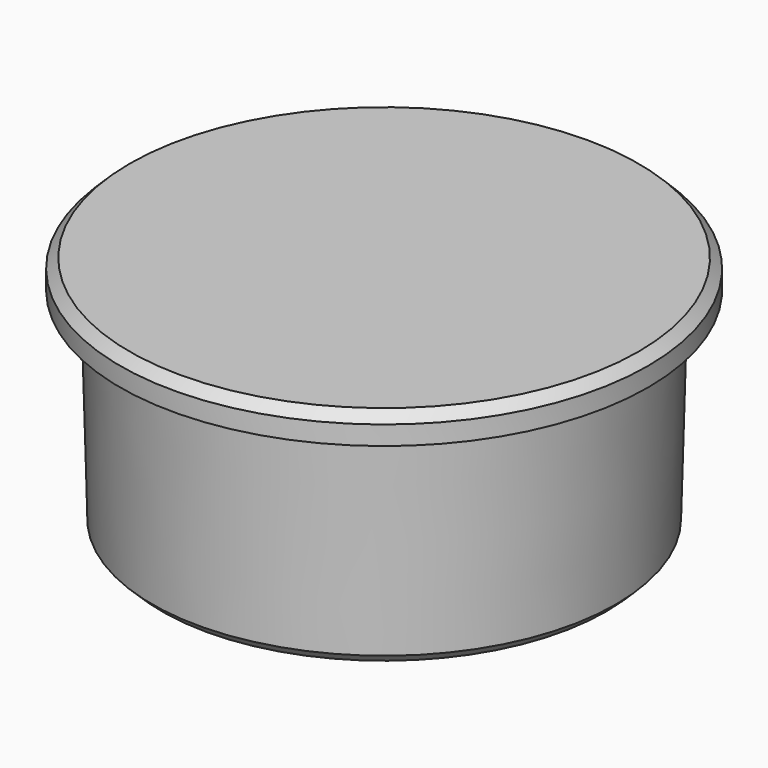
from build123d import *

# Parameters (mm, degrees)
F0_R          = 24.9
F1_DEPTH      = 19.2
F1_TAPER      = 1.5
F1_DEPTH_BACK = 3
F1_TAPER_BACK = -1.5
F2_R          = 27.8
F3_DEPTH      = 3
F4_SIZE       = 1
F5_T          = -2.5
F6_SIZE       = 1


with BuildPart() as f1:
    # F0 (on Top) → F1 (new body, two sides)
    with BuildSketch(Plane.XY) as f1_sk:
        Circle(F0_R)
    extrude(amount=-F1_DEPTH, taper=F1_TAPER)
    extrude(f1_sk.sketch, amount=F1_DEPTH_BACK, taper=F1_TAPER_BACK)

    # F2 (on face) → F3 (join)
    with BuildSketch(Plane.XY.offset(3)):
        Circle(F2_R)
    extrude(amount=F3_DEPTH)

    # F4
    f4_edges = [f1.edges().sort_by_distance(p)[0] for p in [
        (-27.8, 0, 6),
    ]]
    chamfer(f4_edges, length=F4_SIZE)

    # F5
    f5_openings = [f1.faces().sort_by_distance(p)[0] for p in [
        (0, 0, -19.2),
    ]]
    offset(amount=F5_T, openings=f5_openings, kind=Kind.INTERSECTION)

    # F6
    f6_edges = [f1.edges().sort_by_distance(p)[0] for p in [
        (-24.39723, 0, -19.2),
    ]]
    chamfer(f6_edges, length=F6_SIZE)


solid = f1.part
